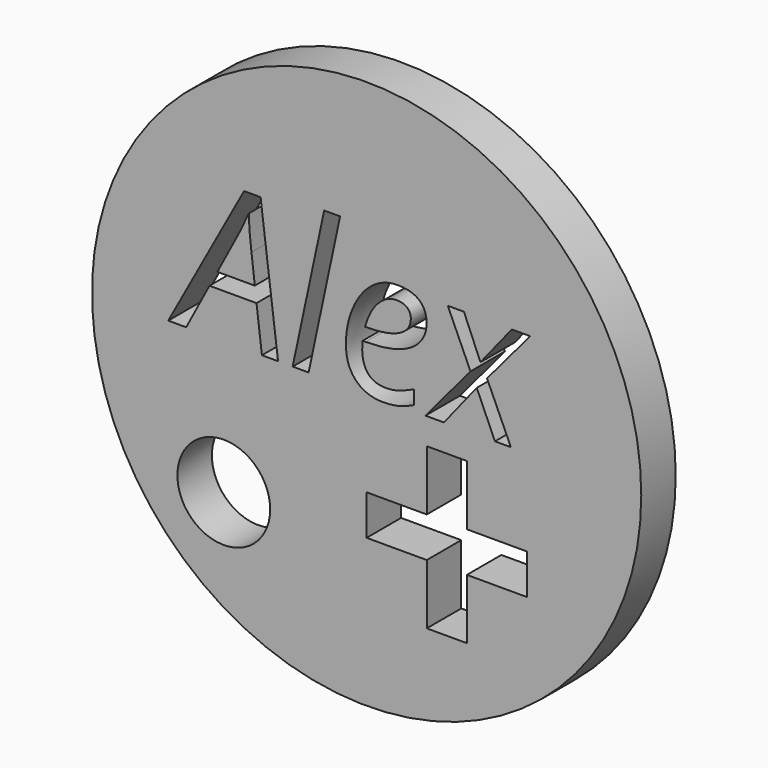
from build123d import *

# Parameters (mm, degrees)
F0_R         = 13.7
F1_DEPTH     = 1.075
F2_R         = 2.3140167045
F3_DEPTH     = 25
F4_TEXT_SIZE = 9.6946798664
F5_DEPTH     = 12.5
F6_W         = 3
F6_H         = 2
F6_W_2       = 2
F6_H_2       = 3
F7_DEPTH     = 25
F8_DEPTH     = 1.075


# Not quite as in the source:
# - Text() gives the source's letters only with a copy of the font that has no kerning and outlines rounded to 1/6400 em; it was checked with that copy


with BuildPart() as f1:
    # F0 (on Front) → F1 (new body, symmetric)
    with BuildSketch(Plane.XZ):
        Circle(F0_R)
    extrude(amount=F1_DEPTH, both=True)

    # F2 (on face) → F3 (cut)
    with BuildSketch(Plane.XZ.offset(1.075)):
        with Locations((-7.1252416819, -6.6389087588)):
            Circle(F2_R)
    extrude(amount=-F3_DEPTH, mode=Mode.SUBTRACT)

    # F4 (on face) → F5 (cut, symmetric)
    with BuildSketch(Plane.XZ.offset(1.075)):
        with Locations((-9.3417329275, 0)):
            Text('Alex', F4_TEXT_SIZE, font='Open Sans', font_style=FontStyle.ITALIC, text_align=(TextAlign.LEFT, TextAlign.BOTTOM))
    extrude(amount=F5_DEPTH, both=True, mode=Mode.SUBTRACT)

    # F6 (on Front) → F7 (cut)
    with BuildSketch(Plane.XZ):
        with Locations((1.5, -5.3193094217)):
            Rectangle(F6_W, F6_H)
        with Locations((4, -2.8193094217)):
            Rectangle(F6_W_2, F6_H_2)
        with Locations((4, -5.3193094217)):
            Rectangle(F6_W_2, F6_H)
        with Locations((6.5, -5.3193094217)):
            Rectangle(F6_W, F6_H)
        with Locations((4, -7.8193094217)):
            Rectangle(F6_W_2, F6_H_2)
    extrude(amount=-F7_DEPTH, mode=Mode.SUBTRACT)

    # F6 (on Front) → F8 (cut, through all)
    with BuildSketch(Plane.XZ):
        with Locations((1.5, -5.3193094217)):
            Rectangle(F6_W, F6_H)
        with Locations((4, -2.8193094217)):
            Rectangle(F6_W_2, F6_H_2)
        with Locations((4, -5.3193094217)):
            Rectangle(F6_W_2, F6_H)
        with Locations((6.5, -5.3193094217)):
            Rectangle(F6_W, F6_H)
        with Locations((4, -7.8193094217)):
            Rectangle(F6_W_2, F6_H_2)
    extrude(amount=F8_DEPTH, mode=Mode.SUBTRACT)


solid = f1.part
